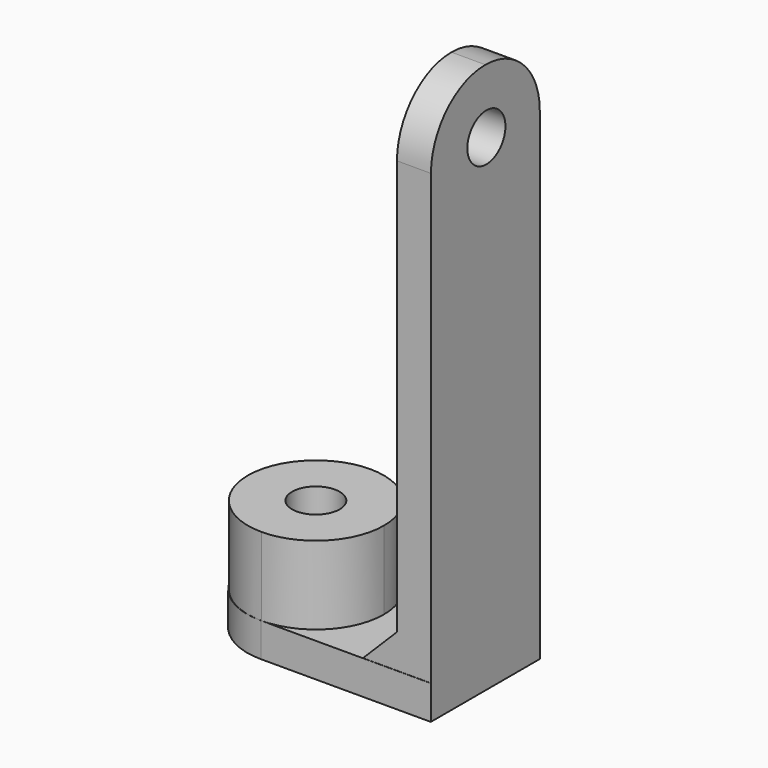
from build123d import *

# Parameters (mm, degrees)
F0_R      = 3.5
F1_DEPTH  = 5
F2_R      = 9.99999
F4_START  = 5
F3_W      = 5
F3_H      = 20
F4_DEPTH  = 76
F5_R      = 3.5
F6_DEPTH  = 79.3
F7_R      = 9.99999
F8_DEPTH  = 16.5
F3_W_2    = 7
F9_DEPTH  = 10
F10_SIZE  = 6.99999
F11_DEPTH = 55.6


# Not quite as in the source:
# - a fillet or chamfer is up to 0.001 mm smaller than in the source, because OpenCascade refuses the exact size


with BuildPart() as f1:
    # F0 (on Top) → F1 (new body)
    with BuildSketch(Plane.XY):
        with BuildLine():
            Line((-36.1016022205, 30.0462352857), (-46.2016022205, 30.0462352857))
            Line((-46.2016022205, 30.0462352857), (-46.2016022205, 10.0462352857))
            Line((-46.2016022205, 10.0462352857), (-36.1016022205, 10.0462352857))
            ThreePointArc((-36.1016022205, 10.0462352857), (-46.1016022205, 20.0462352857), (-36.1016022205, 30.0462352857))
        make_face()
        with BuildLine():
            Line((-11.2016022205, 30.0462352857), (-36.1016022205, 30.0462352857))
            ThreePointArc((-36.1016022205, 30.0462352857), (-29.0305344087, 27.1173030976), (-26.1016022205, 20.0462352857))
            ThreePointArc((-26.1016022205, 20.0462352857), (-29.0305344087, 12.9751674738), (-36.1016022205, 10.0462352857))
            Line((-36.1016022205, 10.0462352857), (-11.2016022205, 10.0462352857))
            Line((-11.2016022205, 10.0462352857), (-11.2016022205, 30.0462352857))
        make_face()
        with BuildLine():
            ThreePointArc((-26.1016022205, 20.0462352857), (-29.0305344087, 27.1173030976), (-36.1016022205, 30.0462352857))
            ThreePointArc((-36.1016022205, 30.0462352857), (-46.1016022205, 20.0462352857), (-36.1016022205, 10.0462352857))
            ThreePointArc((-36.1016022205, 10.0462352857), (-29.0305344087, 12.9751674738), (-26.1016022205, 20.0462352857))
        make_face()
        with Locations((-36.1016022205, 20.0462352857)):
            Circle(F0_R, mode=Mode.SUBTRACT)
    extrude(amount=F1_DEPTH)

    # F2 (radius 10 in the source; OpenCascade refuses exactly that, so slightly less here)
    f2_edges = [f1.edges().sort_by_distance(p)[0] for p in [
        (-46.201602, 30.046235, 2.5),
        (-46.201602, 10.046235, 2.5),
    ]]
    fillet(f2_edges, radius=F2_R)

    # F3 (on Top) → F4 (join)
    with BuildSketch(Plane.XY.offset(F4_START)):
        with Locations((-13.7016022205, 20.0760087371)):
            Rectangle(F3_W, F3_H)
    extrude(amount=F4_DEPTH)

    # F5 (on Right) → F6 (cut)
    with BuildSketch(Plane.YZ):
        with Locations((20.2629771084, 71.5329723358)):
            Circle(F5_R)
    extrude(amount=F6_DEPTH, mode=Mode.SUBTRACT)

    # F7 (radius 10 in the source; OpenCascade refuses exactly that, so slightly less here)
    f7_edges = [f1.edges().sort_by_distance(p)[0] for p in [
        (-13.701602, 10.076009, 81),
        (-13.701602, 30.076009, 81),
    ]]
    fillet(f7_edges, radius=F7_R)

    # F0 (on Top) → F8 (join)
    with BuildSketch(Plane.XY):
        with BuildLine():
            ThreePointArc((-26.1016022205, 20.0462352857), (-29.0305344087, 27.1173030976), (-36.1016022205, 30.0462352857))
            ThreePointArc((-36.1016022205, 30.0462352857), (-46.1016022205, 20.0462352857), (-36.1016022205, 10.0462352857))
            ThreePointArc((-36.1016022205, 10.0462352857), (-29.0305344087, 12.9751674738), (-26.1016022205, 20.0462352857))
        make_face()
        with Locations((-36.1016022205, 20.0462352857)):
            Circle(F0_R, mode=Mode.SUBTRACT)
    extrude(amount=F8_DEPTH)

    # F3 (on Top) → F9 (join)
    with BuildSketch(Plane.XY):
        with Locations((-13.7016022205, 20.0760087371)):
            Rectangle(F3_W, F3_H)
        with Locations((-19.7016022205, 20.0760087371)):
            Rectangle(F3_W_2, F3_H)
    extrude(amount=F9_DEPTH)

    # F10 (size 7 in the source; OpenCascade refuses exactly that, so slightly less here)
    f10_edges = [f1.edges().sort_by_distance(p)[0] for p in [
        (-23.201602, 20.076009, 10),
    ]]
    chamfer(f10_edges, length=F10_SIZE)

    # F5 (on Right) → F11 (cut)
    with BuildSketch(Plane.YZ):
        with Locations((20.2629771084, 71.5329723358)):
            Circle(F5_R)
    extrude(amount=-F11_DEPTH, mode=Mode.SUBTRACT)


solid = f1.part
